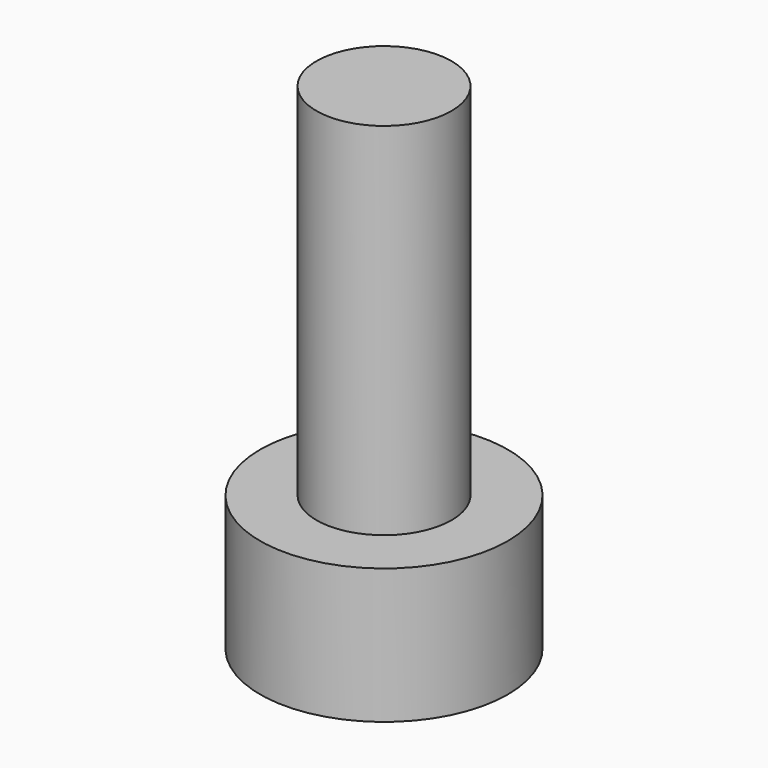
from build123d import *

# Parameters (mm, degrees)
F0_R                   = 2.75
F1_DEPTH               = 3
F2_R                   = 1.5
F3_DEPTH               = 8
F5_DEPTH               = 2.5
F6_DEPTH               = 2.5
DRAFT_F6_DRAFTED_ANGLE = 45


# Not quite as in the source:
# - an extrude with a draft is written as a straight extrude whose walls are then drafted


with BuildPart() as f1:
    # F0 (on Top) → F1 (new body)
    with BuildSketch(Plane.XY):
        Circle(F0_R)
    extrude(amount=F1_DEPTH)

    # F2 (on face) → F3 (join)
    with BuildSketch(Plane.XY.offset(3)):
        Circle(F2_R)
    extrude(amount=F3_DEPTH)

    # F4 (on face) → F5 (cut)
    with BuildSketch(Plane(origin=(0, 0, 0), x_dir=(1, 0, 0), z_dir=(0, 0, -1))):
        Polygon((0.7216878365, -1.25), (1.443375673, 0), (0.7216878365, 1.25), (-0.7216878365, 1.25), (-1.443375673, 0), (-0.7216878365, -1.25), align=None)
    extrude(amount=-F5_DEPTH, mode=Mode.SUBTRACT)


with BuildPart() as f6_drafted:
    # F4 (on face) → F6 (new body)
    with BuildSketch(Plane(origin=(0, 0, 0), x_dir=(1, 0, 0), z_dir=(0, 0, -1))):
        with BuildLine():
            Line((-1.443375673, 0), (-0.7216878365, 1.25))
            ThreePointArc((-0.7216878365, 1.25), (-1.25, 0.7216878365), (-1.443375673, 0))
        make_face()
        with BuildLine():
            Line((-0.7216878365, 1.25), (0.7216878365, 1.25))
            ThreePointArc((0.7216878365, 1.25), (0, 1.443375673), (-0.7216878365, 1.25))
        make_face()
        with BuildLine():
            Line((0.7216878365, 1.25), (1.443375673, 0))
            ThreePointArc((1.443375673, 0), (1.25, 0.7216878365), (0.7216878365, 1.25))
        make_face()
        with BuildLine():
            ThreePointArc((0.7216878365, -1.25), (1.25, -0.7216878365), (1.443375673, 0))
            Line((1.443375673, 0), (0.7216878365, -1.25))
        make_face()
        with BuildLine():
            ThreePointArc((-1.443375673, 0), (-1.25, -0.7216878365), (-0.7216878365, -1.25))
            Line((-0.7216878365, -1.25), (-1.443375673, 0))
        make_face()
        Polygon((0.7216878365, -1.25), (1.443375673, 0), (0.7216878365, 1.25), (-0.7216878365, 1.25), (-1.443375673, 0), (-0.7216878365, -1.25), align=None)
        with BuildLine():
            ThreePointArc((-0.7216878365, -1.25), (0, -1.443375673), (0.7216878365, -1.25))
            Line((0.7216878365, -1.25), (-0.7216878365, -1.25))
        make_face()
    extrude(amount=-F6_DEPTH)

    # draft_F6_drafted
    draft_f6_drafted_walls = [f6_drafted.faces().sort_by_distance(p)[0] for p in [
        (0.7216878365, -1.25, 1.6666666667),
    ]]
    draft(draft_f6_drafted_walls, neutral_plane=Plane.XY, angle=DRAFT_F6_DRAFTED_ANGLE)


with BuildPart() as f1_1:
    add(f1.part)

    # join_F6_drafted: cut F6_drafted
    add(f6_drafted.part, mode=Mode.SUBTRACT)


solid = f1_1.part
